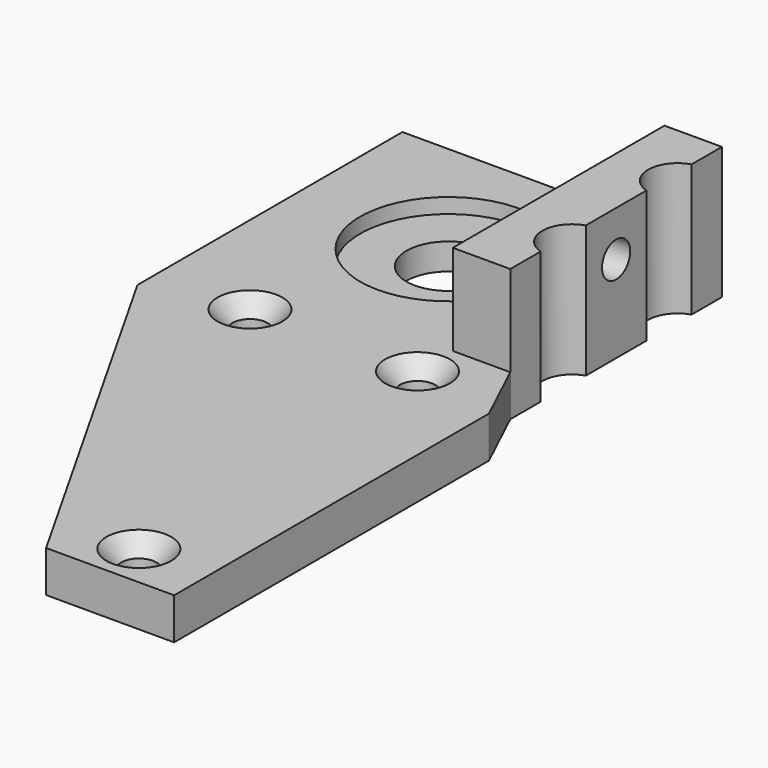
from build123d import *

# Parameters (mm, degrees)
F0_R       = 3.5
F0_R_2     = 10
F0_R_3     = 2
F1_DEPTH   = 4.7
F2_SIZE2   = 1.6781992624
F2_SIZE    = 2
F2_2_SIZE2 = 1.6781992624
F2_2_SIZE  = 2
F2_3_SIZE2 = 1.6781992624
F2_3_SIZE  = 2
F3_DEPTH   = 15
F0_R_4     = 4.75
F4_DEPTH   = 3
F5_R       = 2
F6_DEPTH   = 8


# Not quite as in the source:
# - a feature names something its author has since deleted; it is built from what else it names


with BuildPart() as f1:
    # F0 (on Top) → F1 (new body)
    with BuildSketch(Plane.XY):
        Polygon((-39.2612926662, 18.4351751247), (-14.0709569678, -26), (0.450202167, -26), (0.450202167, 18.6235290021), (-3.0323355459, 26), (-9.549797833, 26), (-9.549797833, 56), (-39.2612926662, 56), align=None)
        with Locations((-7.549797833, -21)):
            Circle(F0_R, mode=Mode.SUBTRACT)
        with Locations((-28.549797833, 21)):
            Circle(F0_R, mode=Mode.SUBTRACT)
        with Locations((-22.049797833, 41)):
            Circle(F0_R_2, mode=Mode.SUBTRACT)
        with Locations((-9.549797833, 21)):
            Circle(F0_R, mode=Mode.SUBTRACT)
        with BuildLine():
            Line((-9.549797833, 26), (-3.0323355459, 26))
            Line((-3.0323355459, 26), (-3.0323355459, 30.2973261729))
            ThreePointArc((-3.0323355459, 30.2973261729), (-5.399797833, 33.5), (-3.0323355459, 36.7026738271))
            Line((-3.0323355459, 36.7026738271), (-3.0323355459, 45.2973261729))
            ThreePointArc((-3.0323355459, 45.2973261729), (-5.399797833, 48.5), (-3.0323355459, 51.7026738271))
            Line((-3.0323355459, 51.7026738271), (-3.0323355459, 56))
            Line((-3.0323355459, 56), (-9.549797833, 56))
            Line((-9.549797833, 56), (-9.549797833, 26))
        make_face()
        with Locations((-28.549797833, 21)):
            Circle(F0_R)
        with Locations((-28.549797833, 21)):
            Circle(F0_R_3, mode=Mode.SUBTRACT)
        with Locations((-9.549797833, 21)):
            Circle(F0_R)
        with Locations((-9.549797833, 21)):
            Circle(F0_R_3, mode=Mode.SUBTRACT)
        with Locations((-7.549797833, -21)):
            Circle(F0_R)
        with Locations((-7.549797833, -21)):
            Circle(F0_R_3, mode=Mode.SUBTRACT)
    extrude(amount=F1_DEPTH)

    # F2
    f2_edges = [f1.edges().sort_by_distance(p)[0] for p in [
        (-30.549798, 21, 4.7),
    ]]
    f2_side = f1.faces().sort_by_distance((-30.549798, 21, 2.35))[0]
    chamfer(f2_edges, length=F2_SIZE, length2=F2_SIZE2, reference=f2_side)

    # F2#2
    f2_2_edges = [f1.edges().sort_by_distance(p)[0] for p in [
        (-11.549798, 21, 4.7),
    ]]
    f2_2_side = f1.faces().sort_by_distance((-11.549798, 21, 2.35))[0]
    chamfer(f2_2_edges, length=F2_2_SIZE, length2=F2_2_SIZE2, reference=f2_2_side)

    # F2#3
    f2_3_edges = [f1.edges().sort_by_distance(p)[0] for p in [
        (-9.549798, -21, 4.7),
    ]]
    f2_3_side = f1.faces().sort_by_distance((-9.549798, -21, 2.35))[0]
    chamfer(f2_3_edges, length=F2_3_SIZE, length2=F2_3_SIZE2, reference=f2_3_side)

    # F0 (on Top) → F3 (join)
    with BuildSketch(Plane.XY):
        with BuildLine():
            Line((-9.549797833, 26), (-3.0323355459, 26))
            Line((-3.0323355459, 26), (-3.0323355459, 30.2973261729))
            ThreePointArc((-3.0323355459, 30.2973261729), (-5.399797833, 33.5), (-3.0323355459, 36.7026738271))
            Line((-3.0323355459, 36.7026738271), (-3.0323355459, 45.2973261729))
            ThreePointArc((-3.0323355459, 45.2973261729), (-5.399797833, 48.5), (-3.0323355459, 51.7026738271))
            Line((-3.0323355459, 51.7026738271), (-3.0323355459, 56))
            Line((-3.0323355459, 56), (-9.549797833, 56))
            Line((-9.549797833, 56), (-9.549797833, 26))
        make_face()
    extrude(amount=F3_DEPTH)

    # F0 (on Top) → F4 (join)
    with BuildSketch(Plane.XY):
        with Locations((-22.049797833, 41)):
            Circle(F0_R_2)
        with Locations((-22.049797833, 41)):
            Circle(F0_R_4, mode=Mode.SUBTRACT)
    extrude(amount=F4_DEPTH)

    # F5 (on face) → F6 (cut)
    with BuildSketch(Plane(origin=(-9.549797833, 0, 0), x_dir=(0, -1, 0), z_dir=(-1, 0, 0))):
        with Locations((-41, 9.85)):
            Circle(F5_R)
    extrude(amount=-F6_DEPTH, mode=Mode.SUBTRACT)


solid = f1.part
